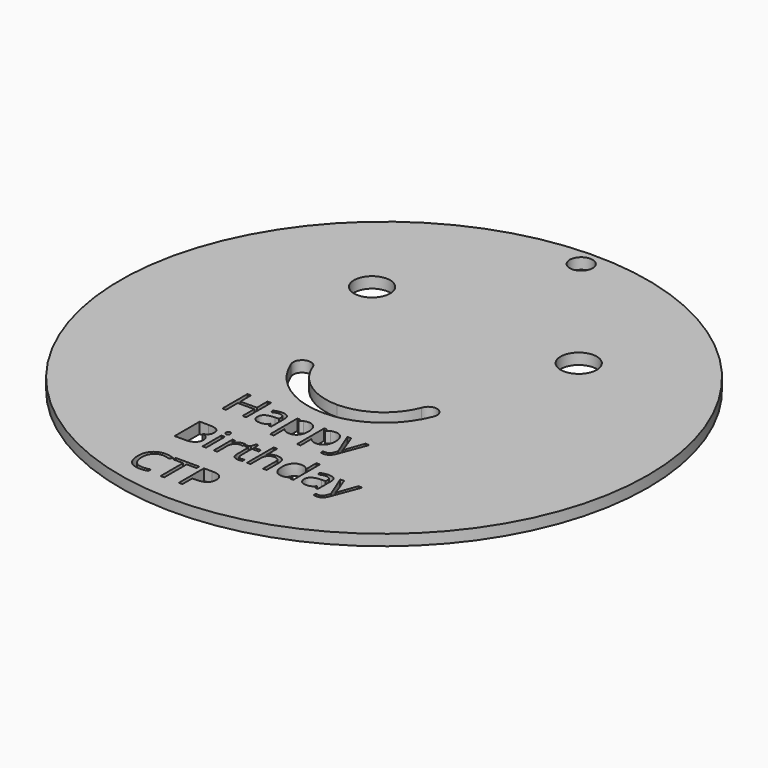
from build123d import *

# Parameters (mm, degrees)
F0_R     = 76.2
F0_W     = 1.0266422647
F0_H     = 6.7750477006
F0_R_2   = 5.2199295035
F0_R_3   = 3.304123166
F1_DEPTH = 3.175


with BuildPart() as f1:
    # F0 (on Top) → F1 (new body)
    with BuildSketch(Plane.XY):
        Circle(F0_R)
        with BuildLine():
            add(Edge.make_bspline(
                [(-13.1552634243, -61.2039017172), (-14.181905689, -60.7232195008), (-15.2085479537, -60.7232195008)],
                knots=[0, 0, 0, 1, 1, 1], degree=2))
            add(Edge.make_bspline(
                [(-15.2085479537, -60.7232195008), (-16.6980693898, -60.7232195008), (-17.5605280168, -61.7152447335)],
                knots=[0, 0, 0, 1, 1, 1], degree=2))
            add(Edge.make_bspline(
                [(-17.5605280168, -61.7152447335), (-18.4229866438, -62.7072699661), (-18.4229866438, -64.4321872201)],
                knots=[0, 0, 0, 1, 1, 1], degree=2))
            add(Edge.make_bspline(
                [(-18.4229866438, -64.4321872201), (-18.4229866438, -66.2045792609), (-17.5911888166, -67.1728671002)],
                knots=[0, 0, 0, 1, 1, 1], degree=2))
            add(Edge.make_bspline(
                [(-17.5911888166, -67.1728671002), (-16.7593909894, -68.1411549394), (-15.2204166504, -68.1411549394)],
                knots=[0, 0, 0, 1, 1, 1], degree=2))
            add(Edge.make_bspline(
                [(-15.2204166504, -68.1411549394), (-14.2748771465, -68.1411549394), (-13.0622919668, -67.8009189673)],
                knots=[0, 0, 0, 1, 1, 1], degree=2))
            Line((-13.0622919668, -67.8009189673), (-13.0622919668, -68.7207429617))
            add(Edge.make_bspline(
                [(-13.0622919668, -68.7207429617), (-14.0018971224, -69.0748257467), (-15.3806440559, -69.0748257467)],
                knots=[0, 0, 0, 1, 1, 1], degree=2))
            add(Edge.make_bspline(
                [(-15.3806440559, -69.0748257467), (-17.3765632179, -69.0748257467), (-18.4615599081, -67.862240567)],
                knots=[0, 0, 0, 1, 1, 1], degree=2))
            add(Edge.make_bspline(
                [(-18.4615599081, -67.862240567), (-19.5465565983, -66.6496553873), (-19.5465565983, -64.4183404073)],
                knots=[0, 0, 0, 1, 1, 1], degree=2))
            add(Edge.make_bspline(
                [(-19.5465565983, -64.4183404073), (-19.5465565983, -63.0217904287), (-19.0243339434, -61.9714107706)],
                knots=[0, 0, 0, 1, 1, 1], degree=2))
            add(Edge.make_bspline(
                [(-19.0243339434, -61.9714107706), (-18.5021112885, -60.9210311125), (-17.5160204042, -60.3523227289)],
                knots=[0, 0, 0, 1, 1, 1], degree=2))
            add(Edge.make_bspline(
                [(-17.5160204042, -60.3523227289), (-16.5299295199, -59.7836143452), (-15.1947011409, -59.7836143452)],
                knots=[0, 0, 0, 1, 1, 1], degree=2))
            add(Edge.make_bspline(
                [(-15.1947011409, -59.7836143452), (-13.7744137689, -59.7836143452), (-12.710187298, -60.3018807679)],
                knots=[0, 0, 0, 1, 1, 1], degree=2))
            Line((-12.710187298, -60.3018807679), (-13.1552634243, -61.2039017172))
        make_face(mode=Mode.SUBTRACT)
        Polygon((-8.3088789377, -60.8458627001), (-8.3088789377, -68.9502044313), (-9.3592585958, -68.9502044313), (-9.3592585958, -60.8458627001), (-12.2215926171, -60.8458627001), (-12.2215926171, -59.9121918928), (-5.4465449165, -59.9121918928), (-5.4465449165, -60.8458627001), align=None, mode=Mode.SUBTRACT)
        with BuildLine():
            add(Edge.make_bspline(
                [(-1.7415334294, -59.9121918928), (1.6450013629, -59.9121918928), (1.6450013629, -62.5450644445)],
                knots=[0, 0, 0, 1, 1, 1], degree=2))
            add(Edge.make_bspline(
                [(1.6450013629, -62.5450644445), (1.6450013629, -63.9178770297), (0.7083633815, -64.6567033994)],
                knots=[0, 0, 0, 1, 1, 1], degree=2))
            add(Edge.make_bspline(
                [(0.7083633815, -64.6567033994), (-0.2282745999, -65.3955297691), (-1.970994899, -65.3955297691)],
                knots=[0, 0, 0, 1, 1, 1], degree=2))
            Line((-1.970994899, -65.3955297691), (-3.0352213699, -65.3955297691))
            Line((-3.0352213699, -65.3955297691), (-3.0352213699, -68.9502044313))
            Line((-3.0352213699, -68.9502044313), (-4.085601028, -68.9502044313))
            Line((-4.085601028, -68.9502044313), (-4.085601028, -59.9121918928))
            Line((-4.085601028, -59.9121918928), (-1.7415334294, -59.9121918928))
        make_face(mode=Mode.SUBTRACT)
        with Locations((-10.5154674662, -48.3451578988)):
            Rectangle(F0_W, F0_H, mode=Mode.SUBTRACT)
        with BuildLine():
            add(Edge.make_bspline(
                [(-5.9034897395, -45.1920408084), (-5.371376504, -44.8330127331), (-4.7344231144, -44.8330127331)],
                knots=[0, 0, 0, 1, 1, 1], degree=2))
            add(Edge.make_bspline(
                [(-4.7344231144, -44.8330127331), (-4.2834126397, -44.8330127331), (-3.9253736225, -44.9081811456)],
                knots=[0, 0, 0, 1, 1, 1], degree=2))
            Line((-3.9253736225, -44.9081811456), (-4.0677979829, -45.8596549979))
            add(Edge.make_bspline(
                [(-4.0677979829, -45.8596549979), (-4.4871585997, -45.7666835404), (-4.8095915268, -45.7666835404)],
                knots=[0, 0, 0, 1, 1, 1], degree=2))
            add(Edge.make_bspline(
                [(-4.8095915268, -45.7666835404), (-5.6324878315, -45.7666835404), (-6.216032086, -46.4342977298)],
                knots=[0, 0, 0, 1, 1, 1], degree=2))
            add(Edge.make_bspline(
                [(-6.216032086, -46.4342977298), (-6.7995763405, -47.1019119193), (-6.7995763405, -48.0969043262)],
                knots=[0, 0, 0, 1, 1, 1], degree=2))
            Line((-6.7995763405, -48.0969043262), (-6.7995763405, -51.7326817492))
            Line((-6.7995763405, -51.7326817492), (-7.8262186052, -51.7326817492))
            Line((-7.8262186052, -51.7326817492), (-7.8262186052, -44.9576340485))
            Line((-7.8262186052, -44.9576340485), (-6.9795849071, -44.9576340485))
            Line((-6.9795849071, -44.9576340485), (-6.8608979401, -46.2117596667))
            Line((-6.8608979401, -46.2117596667), (-6.8114450372, -46.2117596667))
            add(Edge.make_bspline(
                [(-6.8114450372, -46.2117596667), (-6.435602975, -45.5510688836), (-5.9034897395, -45.1920408084)],
                knots=[0, 0, 0, 1, 1, 1], degree=2))
        make_face(mode=Mode.SUBTRACT)
        with BuildLine():
            Line((-19.0777430785, -51.7326817492), (-19.0777430785, -42.6946692107))
            Line((-19.0777430785, -42.6946692107), (-16.5239951715, -42.6946692107))
            add(Edge.make_bspline(
                [(-16.5239951715, -42.6946692107), (-14.7258876212, -42.6946692107), (-13.9217834196, -43.2327167945)],
                knots=[0, 0, 0, 1, 1, 1], degree=2))
            add(Edge.make_bspline(
                [(-13.9217834196, -43.2327167945), (-13.1176792181, -43.7707643783), (-13.1176792181, -44.931918539)],
                knots=[0, 0, 0, 1, 1, 1], degree=2))
            add(Edge.make_bspline(
                [(-13.1176792181, -44.931918539), (-13.1176792181, -45.7370117986), (-13.5657225186, -46.2592344535)],
                knots=[0, 0, 0, 1, 1, 1], degree=2))
            add(Edge.make_bspline(
                [(-13.5657225186, -46.2592344535), (-14.0137658191, -46.7814571084), (-14.87424633, -46.9357501655)],
                knots=[0, 0, 0, 1, 1, 1], degree=2))
            Line((-14.87424633, -46.9357501655), (-14.87424633, -46.9970717651))
            add(Edge.make_bspline(
                [(-14.87424633, -46.9970717651), (-12.8150274522, -47.3491764339), (-12.8150274522, -49.1611307971)],
                knots=[0, 0, 0, 1, 1, 1], degree=2))
            add(Edge.make_bspline(
                [(-12.8150274522, -49.1611307971), (-12.8150274522, -50.3717378607), (-13.6339675246, -51.0522098049)],
                knots=[0, 0, 0, 1, 1, 1], degree=2))
            add(Edge.make_bspline(
                [(-13.6339675246, -51.0522098049), (-14.4529075971, -51.7326817492), (-15.9246259881, -51.7326817492)],
                knots=[0, 0, 0, 1, 1, 1], degree=2))
            Line((-15.9246259881, -51.7326817492), (-19.0777430785, -51.7326817492))
        make_face(mode=Mode.SUBTRACT)
        with BuildLine():
            add(Edge.make_bspline(
                [(-10.9427405475, -43.6382305985), (-11.1158257077, -43.4681126124), (-11.1158257077, -43.121942292)],
                knots=[0, 0, 0, 1, 1, 1], degree=2))
            add(Edge.make_bspline(
                [(-11.1158257077, -43.121942292), (-11.1158257077, -42.7698376231), (-10.9427405475, -42.6056539854)],
                knots=[0, 0, 0, 1, 1, 1], degree=2))
            add(Edge.make_bspline(
                [(-10.9427405475, -42.6056539854), (-10.7696553873, -42.4414703477), (-10.5085440598, -42.4414703477)],
                knots=[0, 0, 0, 1, 1, 1], degree=2))
            add(Edge.make_bspline(
                [(-10.5085440598, -42.4414703477), (-10.2612795452, -42.4414703477), (-10.0822600366, -42.6086211596)],
                knots=[0, 0, 0, 1, 1, 1], degree=2))
            add(Edge.make_bspline(
                [(-10.0822600366, -42.6086211596), (-9.903240528, -42.7757719715), (-9.903240528, -43.121942292)],
                knots=[0, 0, 0, 1, 1, 1], degree=2))
            add(Edge.make_bspline(
                [(-9.903240528, -43.121942292), (-9.903240528, -43.4681126124), (-10.0822600366, -43.6382305985)],
                knots=[0, 0, 0, 1, 1, 1], degree=2))
            add(Edge.make_bspline(
                [(-10.0822600366, -43.6382305985), (-10.2612795452, -43.8083485846), (-10.5085440598, -43.8083485846)],
                knots=[0, 0, 0, 1, 1, 1], degree=2))
            add(Edge.make_bspline(
                [(-10.5085440598, -43.8083485846), (-10.7696553873, -43.8083485846), (-10.9427405475, -43.6382305985)],
                knots=[0, 0, 0, 1, 1, 1], degree=2))
        make_face(mode=Mode.SUBTRACT)
        with BuildLine():
            add(Edge.make_bspline(
                [(-1.2667855613, -50.681313033), (-0.9760024921, -51.0086912503), (-0.4696047662, -51.0086912503)],
                knots=[0, 0, 0, 1, 1, 1], degree=2))
            add(Edge.make_bspline(
                [(-0.4696047662, -51.0086912503), (-0.196624742, -51.0086912503), (0.0565741209, -50.969128928)],
                knots=[0, 0, 0, 1, 1, 1], degree=2))
            add(Edge.make_bspline(
                [(0.0565741209, -50.969128928), (0.3097729839, -50.9295666057), (0.4581316927, -50.8860480511)],
                knots=[0, 0, 0, 1, 1, 1], degree=2))
            Line((0.4581316927, -50.8860480511), (0.4581316927, -51.6713601495))
            add(Edge.make_bspline(
                [(0.4581316927, -51.6713601495), (0.2919699389, -51.7504847942), (-0.0324411043, -51.8038939294)],
                knots=[0, 0, 0, 1, 1, 1], degree=2))
            add(Edge.make_bspline(
                [(-0.0324411043, -51.8038939294), (-0.3568521475, -51.8573030645), (-0.6179634749, -51.8573030645)],
                knots=[0, 0, 0, 1, 1, 1], degree=2))
            add(Edge.make_bspline(
                [(-0.6179634749, -51.8573030645), (-2.5822327791, -51.8573030645), (-2.5822327791, -49.7862154901)],
                knots=[0, 0, 0, 1, 1, 1], degree=2))
            Line((-2.5822327791, -49.7862154901), (-2.5822327791, -45.7548148437))
            Line((-2.5822327791, -45.7548148437), (-3.5534877925, -45.7548148437))
            Line((-3.5534877925, -45.7548148437), (-3.5534877925, -45.2602858144))
            Line((-3.5534877925, -45.2602858144), (-2.5822327791, -44.8330127331))
            Line((-2.5822327791, -44.8330127331), (-2.1510034656, -43.3870098516))
            Line((-2.1510034656, -43.3870098516), (-1.5575686305, -43.3870098516))
            Line((-1.5575686305, -43.3870098516), (-1.5575686305, -44.9576340485))
            Line((-1.5575686305, -44.9576340485), (0.4086787898, -44.9576340485))
            Line((0.4086787898, -44.9576340485), (0.4086787898, -45.7548148437))
            Line((0.4086787898, -45.7548148437), (-1.5575686305, -45.7548148437))
            Line((-1.5575686305, -45.7548148437), (-1.5575686305, -49.7426969355))
            add(Edge.make_bspline(
                [(-1.5575686305, -49.7426969355), (-1.5575686305, -50.3539348156), (-1.2667855613, -50.681313033)],
                knots=[0, 0, 0, 1, 1, 1], degree=2))
        make_face(mode=Mode.SUBTRACT)
        Polygon((-12.2156582688, -25.4771465286), (-12.2156582688, -34.515159067), (-13.2660379269, -34.515159067), (-13.2660379269, -30.2622094155), (-18.0273634204, -30.2622094155), (-18.0273634204, -34.515159067), (-19.0777430785, -34.515159067), (-19.0777430785, -25.4771465286), (-18.0273634204, -25.4771465286), (-18.0273634204, -29.32260426), (-13.2660379269, -29.32260426), (-13.2660379269, -25.4771465286), align=None, mode=Mode.SUBTRACT)
        with BuildLine():
            Line((-4.9638845839, -34.515159067), (-5.725459289, -34.515159067))
            Line((-5.725459289, -34.515159067), (-5.929205249, -33.5498384019))
            Line((-5.929205249, -33.5498384019), (-5.9786581519, -33.5498384019))
            add(Edge.make_bspline(
                [(-5.9786581519, -33.5498384019), (-6.4850558779, -34.1867917916), (-6.9884864297, -34.413286087)],
                knots=[0, 0, 0, 1, 1, 1], degree=2))
            add(Edge.make_bspline(
                [(-6.9884864297, -34.413286087), (-7.4919169814, -34.6397803824), (-8.2475573381, -34.6397803824)],
                knots=[0, 0, 0, 1, 1, 1], degree=2))
            add(Edge.make_bspline(
                [(-8.2475573381, -34.6397803824), (-9.2544184416, -34.6397803824), (-9.8260939995, -34.1195358436)],
                knots=[0, 0, 0, 1, 1, 1], degree=2))
            add(Edge.make_bspline(
                [(-9.8260939995, -34.1195358436), (-10.3977695573, -33.5992913049), (-10.3977695573, -32.6418831042)],
                knots=[0, 0, 0, 1, 1, 1], degree=2))
            add(Edge.make_bspline(
                [(-10.3977695573, -32.6418831042), (-10.3977695573, -30.5905766909), (-7.1160749192, -30.4916708851)],
                knots=[0, 0, 0, 1, 1, 1], degree=2))
            Line((-7.1160749192, -30.4916708851), (-5.9667894552, -30.4540866789))
            Line((-5.9667894552, -30.4540866789), (-5.9667894552, -30.032747946))
            add(Edge.make_bspline(
                [(-5.9667894552, -30.032747946), (-5.9667894552, -29.2355671508), (-6.3090035435, -28.8557688564)],
                knots=[0, 0, 0, 1, 1, 1], degree=2))
            add(Edge.make_bspline(
                [(-6.3090035435, -28.8557688564), (-6.6512176317, -28.4759705619), (-7.4068579884, -28.4759705619)],
                knots=[0, 0, 0, 1, 1, 1], degree=2))
            add(Edge.make_bspline(
                [(-7.4068579884, -28.4759705619), (-8.2534916865, -28.4759705619), (-9.3216743896, -28.9942369845)],
                knots=[0, 0, 0, 1, 1, 1], degree=2))
            Line((-9.3216743896, -28.9942369845), (-9.6381729683, -28.2089248861))
            add(Edge.make_bspline(
                [(-9.6381729683, -28.2089248861), (-9.1377095907, -27.9379229781), (-8.5413075815, -27.783629921)],
                knots=[0, 0, 0, 1, 1, 1], degree=2))
            add(Edge.make_bspline(
                [(-8.5413075815, -27.783629921), (-7.9449055722, -27.6293368638), (-7.3435582727, -27.6293368638)],
                knots=[0, 0, 0, 1, 1, 1], degree=2))
            add(Edge.make_bspline(
                [(-7.3435582727, -27.6293368638), (-6.1329512091, -27.6293368638), (-5.5484178965, -28.1663953896)],
                knots=[0, 0, 0, 1, 1, 1], degree=2))
            add(Edge.make_bspline(
                [(-5.5484178965, -28.1663953896), (-4.9638845839, -28.7034539153), (-4.9638845839, -29.8903235855)],
                knots=[0, 0, 0, 1, 1, 1], degree=2))
            Line((-4.9638845839, -29.8903235855), (-4.9638845839, -34.515159067))
        make_face(mode=Mode.SUBTRACT)
        with BuildLine():
            Line((7.4745095596, -51.7326817492), (6.4478672949, -51.7326817492))
            Line((6.4478672949, -51.7326817492), (6.4478672949, -47.3491764339))
            add(Edge.make_bspline(
                [(6.4478672949, -47.3491764339), (6.4478672949, -46.522323897), (6.0710361746, -46.1138429189)],
                knots=[0, 0, 0, 1, 1, 1], degree=2))
            add(Edge.make_bspline(
                [(6.0710361746, -46.1138429189), (5.6942050543, -45.7053619407), (4.8891117947, -45.7053619407)],
                knots=[0, 0, 0, 1, 1, 1], degree=2))
            add(Edge.make_bspline(
                [(4.8891117947, -45.7053619407), (3.8209290915, -45.7053619407), (3.3293672365, -46.2869280791)],
                knots=[0, 0, 0, 1, 1, 1], degree=2))
            add(Edge.make_bspline(
                [(3.3293672365, -46.2869280791), (2.8378053814, -46.8684942175), (2.8378053814, -48.1898757837)],
                knots=[0, 0, 0, 1, 1, 1], degree=2))
            Line((2.8378053814, -48.1898757837), (2.8378053814, -51.7326817492))
            Line((2.8378053814, -51.7326817492), (1.8111631167, -51.7326817492))
            Line((1.8111631167, -51.7326817492), (1.8111631167, -42.1131030723))
            Line((1.8111631167, -42.1131030723), (2.8378053814, -42.1131030723))
            Line((2.8378053814, -42.1131030723), (2.8378053814, -45.0248899965))
            add(Edge.make_bspline(
                [(2.8378053814, -45.0248899965), (2.8378053814, -45.5510688836), (2.7883524785, -45.8972392041)],
                knots=[0, 0, 0, 1, 1, 1], degree=2))
            Line((2.7883524785, -45.8972392041), (2.8496740781, -45.8972392041))
            add(Edge.make_bspline(
                [(2.8496740781, -45.8972392041), (3.152325844, -45.4086445232), (3.7121327051, -45.1277520346)],
                knots=[0, 0, 0, 1, 1, 1], degree=2))
            add(Edge.make_bspline(
                [(3.7121327051, -45.1277520346), (4.2719395662, -44.846859546), (4.9880176006, -44.846859546)],
                knots=[0, 0, 0, 1, 1, 1], degree=2))
            add(Edge.make_bspline(
                [(4.9880176006, -44.846859546), (6.230274522, -44.846859546), (6.8523920408, -45.4373272069)],
                knots=[0, 0, 0, 1, 1, 1], degree=2))
            add(Edge.make_bspline(
                [(6.8523920408, -45.4373272069), (7.4745095596, -46.0277948678), (7.4745095596, -47.3135703438)],
                knots=[0, 0, 0, 1, 1, 1], degree=2))
            Line((7.4745095596, -47.3135703438), (7.4745095596, -51.7326817492))
        make_face(mode=Mode.SUBTRACT)
        with BuildLine():
            Line((14.3286819049, -51.7326817492), (14.1921918928, -50.8247264515))
            Line((14.1921918928, -50.8247264515), (14.1368046416, -50.8247264515))
            add(Edge.make_bspline(
                [(14.1368046416, -50.8247264515), (13.4266609556, -51.8573030645), (12.0103298158, -51.8573030645)],
                knots=[0, 0, 0, 1, 1, 1], degree=2))
            add(Edge.make_bspline(
                [(12.0103298158, -51.8573030645), (10.6810357852, -51.8573030645), (9.9422094155, -50.9483587088)],
                knots=[0, 0, 0, 1, 1, 1], degree=2))
            add(Edge.make_bspline(
                [(9.9422094155, -50.9483587088), (9.2033830458, -50.039414353), (9.2033830458, -48.3639500019)],
                knots=[0, 0, 0, 1, 1, 1], degree=2))
            add(Edge.make_bspline(
                [(9.2033830458, -48.3639500019), (9.2033830458, -46.6884856509), (9.9451765897, -45.760749192)],
                knots=[0, 0, 0, 1, 1, 1], degree=2))
            add(Edge.make_bspline(
                [(9.9451765897, -45.760749192), (10.6869701336, -44.8330127331), (12.0103298158, -44.8330127331)],
                knots=[0, 0, 0, 1, 1, 1], degree=2))
            add(Edge.make_bspline(
                [(12.0103298158, -44.8330127331), (13.3890767493, -44.8330127331), (14.1249359449, -45.8359176045)],
                knots=[0, 0, 0, 1, 1, 1], degree=2))
            Line((14.1249359449, -45.8359176045), (14.2060387057, -45.8359176045))
            Line((14.2060387057, -45.8359176045), (14.1625201511, -45.3473229236))
            Line((14.1625201511, -45.3473229236), (14.1368046416, -44.8705969394))
            Line((14.1368046416, -44.8705969394), (14.1368046416, -42.1131030723))
            Line((14.1368046416, -42.1131030723), (15.1634469063, -42.1131030723))
            Line((15.1634469063, -42.1131030723), (15.1634469063, -51.7326817492))
            Line((15.1634469063, -51.7326817492), (14.3286819049, -51.7326817492))
        make_face(mode=Mode.SUBTRACT)
        with BuildLine():
            Line((22.2668618823, -51.7326817492), (21.5052871773, -51.7326817492))
            Line((21.5052871773, -51.7326817492), (21.3015412172, -50.7673610841))
            Line((21.3015412172, -50.7673610841), (21.2520883143, -50.7673610841))
            add(Edge.make_bspline(
                [(21.2520883143, -50.7673610841), (20.7456905884, -51.4043144737), (20.2422600366, -51.6308087691)],
                knots=[0, 0, 0, 1, 1, 1], degree=2))
            add(Edge.make_bspline(
                [(20.2422600366, -51.6308087691), (19.7388294848, -51.8573030645), (18.9831891281, -51.8573030645)],
                knots=[0, 0, 0, 1, 1, 1], degree=2))
            add(Edge.make_bspline(
                [(18.9831891281, -51.8573030645), (17.9763280246, -51.8573030645), (17.4046524668, -51.3370585258)],
                knots=[0, 0, 0, 1, 1, 1], degree=2))
            add(Edge.make_bspline(
                [(17.4046524668, -51.3370585258), (16.832976909, -50.816813987), (16.832976909, -49.8594057864)],
                knots=[0, 0, 0, 1, 1, 1], degree=2))
            add(Edge.make_bspline(
                [(16.832976909, -49.8594057864), (16.832976909, -47.8080993731), (20.1146715471, -47.7091935672)],
                knots=[0, 0, 0, 1, 1, 1], degree=2))
            Line((20.1146715471, -47.7091935672), (21.263957011, -47.671609361))
            Line((21.263957011, -47.671609361), (21.263957011, -47.2502706281))
            add(Edge.make_bspline(
                [(21.263957011, -47.2502706281), (21.263957011, -46.453089833), (20.9217429228, -46.0732915385)],
                knots=[0, 0, 0, 1, 1, 1], degree=2))
            add(Edge.make_bspline(
                [(20.9217429228, -46.0732915385), (20.5795288345, -45.693493244), (19.8238884779, -45.693493244)],
                knots=[0, 0, 0, 1, 1, 1], degree=2))
            add(Edge.make_bspline(
                [(19.8238884779, -45.693493244), (18.9772547798, -45.693493244), (17.9090720766, -46.2117596667)],
                knots=[0, 0, 0, 1, 1, 1], degree=2))
            Line((17.9090720766, -46.2117596667), (17.5925734979, -45.4264475682))
            add(Edge.make_bspline(
                [(17.5925734979, -45.4264475682), (18.0930368755, -45.1554456602), (18.6894388848, -45.0011526031)],
                knots=[0, 0, 0, 1, 1, 1], degree=2))
            add(Edge.make_bspline(
                [(18.6894388848, -45.0011526031), (19.285840894, -44.846859546), (19.8871881936, -44.846859546)],
                knots=[0, 0, 0, 1, 1, 1], degree=2))
            add(Edge.make_bspline(
                [(19.8871881936, -44.846859546), (21.0977952572, -44.846859546), (21.6823285698, -45.3839180717)],
                knots=[0, 0, 0, 1, 1, 1], degree=2))
            add(Edge.make_bspline(
                [(21.6823285698, -45.3839180717), (22.2668618823, -45.9209765975), (22.2668618823, -47.1078462677)],
                knots=[0, 0, 0, 1, 1, 1], degree=2))
            Line((22.2668618823, -47.1078462677), (22.2668618823, -51.7326817492))
        make_face(mode=Mode.SUBTRACT)
        with BuildLine():
            Line((26.0371512013, -51.7702659554), (23.3033947276, -44.9576340485))
            Line((23.3033947276, -44.9576340485), (24.4052054048, -44.9576340485))
            Line((24.4052054048, -44.9576340485), (25.8887924925, -48.820894825))
            add(Edge.make_bspline(
                [(25.8887924925, -48.820894825), (26.3754090573, -50.1442545072), (26.4940960243, -50.731754994)],
                knots=[0, 0, 0, 1, 1, 1], degree=2))
            Line((26.4940960243, -50.731754994), (26.5435489272, -50.731754994))
            add(Edge.make_bspline(
                [(26.5435489272, -50.731754994), (26.6226735719, -50.4152564152), (26.8798286671, -49.6517035941)],
                knots=[0, 0, 0, 1, 1, 1], degree=2))
            add(Edge.make_bspline(
                [(26.8798286671, -49.6517035941), (27.1369837623, -48.8881507729), (28.5592492504, -44.9576340485)],
                knots=[0, 0, 0, 1, 1, 1], degree=2))
            Line((28.5592492504, -44.9576340485), (29.6590818115, -44.9576340485))
            Line((29.6590818115, -44.9576340485), (26.7472948873, -52.6722869047))
            add(Edge.make_bspline(
                [(26.7472948873, -52.6722869047), (26.3140874577, -53.8156380203), (25.7364775515, -54.2953311787)],
                knots=[0, 0, 0, 1, 1, 1], degree=2))
            add(Edge.make_bspline(
                [(25.7364775515, -54.2953311787), (25.1588676453, -54.7750243371), (24.3181682956, -54.7750243371)],
                knots=[0, 0, 0, 1, 1, 1], degree=2))
            add(Edge.make_bspline(
                [(24.3181682956, -54.7750243371), (23.8473766598, -54.7750243371), (23.3904318368, -54.6682060667)],
                knots=[0, 0, 0, 1, 1, 1], degree=2))
            Line((23.3904318368, -54.6682060667), (23.3904318368, -53.8472878782))
            add(Edge.make_bspline(
                [(23.3904318368, -53.8472878782), (23.7306678089, -53.9204781745), (24.1500284257, -53.9204781745)],
                knots=[0, 0, 0, 1, 1, 1], degree=2))
            add(Edge.make_bspline(
                [(24.1500284257, -53.9204781745), (25.2083205483, -53.9204781745), (25.6593310229, -52.7336085043)],
                knots=[0, 0, 0, 1, 1, 1], degree=2))
            Line((25.6593310229, -52.7336085043), (26.0371512013, -51.7702659554))
        make_face(mode=Mode.SUBTRACT)
        with BuildLine():
            add(Edge.make_bspline(
                [(2.3699809197, -33.7150110977), (1.6252202017, -34.6397803824), (0.3018605195, -34.6397803824)],
                knots=[0, 0, 0, 1, 1, 1], degree=2))
            add(Edge.make_bspline(
                [(0.3018605195, -34.6397803824), (-0.3608083797, -34.6397803824), (-0.9077574861, -34.3954830419)],
                knots=[0, 0, 0, 1, 1, 1], degree=2))
            add(Edge.make_bspline(
                [(-0.9077574861, -34.3954830419), (-1.4547065924, -34.1511857015), (-1.8246143063, -33.6428098594)],
                knots=[0, 0, 0, 1, 1, 1], degree=2))
            Line((-1.8246143063, -33.6428098594), (-1.8997827187, -33.6428098594))
            add(Edge.make_bspline(
                [(-1.8997827187, -33.6428098594), (-1.8246143063, -34.2362446945), (-1.8246143063, -34.76835793)],
                knots=[0, 0, 0, 1, 1, 1], degree=2))
            Line((-1.8246143063, -34.76835793), (-1.8246143063, -37.5575016549))
            Line((-1.8246143063, -37.5575016549), (-2.851256571, -37.5575016549))
            Line((-2.851256571, -37.5575016549), (-2.851256571, -27.7401113664))
            Line((-2.851256571, -27.7401113664), (-2.0164915696, -27.7401113664))
            Line((-2.0164915696, -27.7401113664), (-1.8740672092, -28.6678478252))
            Line((-1.8740672092, -28.6678478252), (-1.8246143063, -28.6678478252))
            add(Edge.make_bspline(
                [(-1.8246143063, -28.6678478252), (-1.4289910829, -28.1100190803), (-0.9038012538, -27.8627545656)],
                knots=[0, 0, 0, 1, 1, 1], degree=2))
            add(Edge.make_bspline(
                [(-0.9038012538, -27.8627545656), (-0.3786114248, -27.615490051), (0.3018605195, -27.615490051)],
                knots=[0, 0, 0, 1, 1, 1], degree=2))
            add(Edge.make_bspline(
                [(0.3018605195, -27.615490051), (1.6489575951, -27.615490051), (2.3818496164, -28.5372921615)],
                knots=[0, 0, 0, 1, 1, 1], degree=2))
            add(Edge.make_bspline(
                [(2.3818496164, -28.5372921615), (3.1147416378, -29.459094272), (3.1147416378, -31.1207118103)],
                knots=[0, 0, 0, 1, 1, 1], degree=2))
            add(Edge.make_bspline(
                [(3.1147416378, -31.1207118103), (3.1147416378, -32.790241813), (2.3699809197, -33.7150110977)],
                knots=[0, 0, 0, 1, 1, 1], degree=2))
        make_face(mode=Mode.SUBTRACT)
        with BuildLine():
            add(Edge.make_bspline(
                [(10.1281523305, -33.7150110977), (9.3833916125, -34.6397803824), (8.0600319302, -34.6397803824)],
                knots=[0, 0, 0, 1, 1, 1], degree=2))
            add(Edge.make_bspline(
                [(8.0600319302, -34.6397803824), (7.397363031, -34.6397803824), (6.8504139247, -34.3954830419)],
                knots=[0, 0, 0, 1, 1, 1], degree=2))
            add(Edge.make_bspline(
                [(6.8504139247, -34.3954830419), (6.3034648183, -34.1511857015), (5.9335571045, -33.6428098594)],
                knots=[0, 0, 0, 1, 1, 1], degree=2))
            Line((5.9335571045, -33.6428098594), (5.858388692, -33.6428098594))
            add(Edge.make_bspline(
                [(5.858388692, -33.6428098594), (5.9335571045, -34.2362446945), (5.9335571045, -34.76835793)],
                knots=[0, 0, 0, 1, 1, 1], degree=2))
            Line((5.9335571045, -34.76835793), (5.9335571045, -37.5575016549))
            Line((5.9335571045, -37.5575016549), (4.9069148398, -37.5575016549))
            Line((4.9069148398, -37.5575016549), (4.9069148398, -27.7401113664))
            Line((4.9069148398, -27.7401113664), (5.7416798411, -27.7401113664))
            Line((5.7416798411, -27.7401113664), (5.8841042015, -28.6678478252))
            Line((5.8841042015, -28.6678478252), (5.9335571045, -28.6678478252))
            add(Edge.make_bspline(
                [(5.9335571045, -28.6678478252), (6.3291803279, -28.1100190803), (6.8543701569, -27.8627545656)],
                knots=[0, 0, 0, 1, 1, 1], degree=2))
            add(Edge.make_bspline(
                [(6.8543701569, -27.8627545656), (7.379559986, -27.615490051), (8.0600319302, -27.615490051)],
                knots=[0, 0, 0, 1, 1, 1], degree=2))
            add(Edge.make_bspline(
                [(8.0600319302, -27.615490051), (9.4071290059, -27.615490051), (10.1400210272, -28.5372921615)],
                knots=[0, 0, 0, 1, 1, 1], degree=2))
            add(Edge.make_bspline(
                [(10.1400210272, -28.5372921615), (10.8729130486, -29.459094272), (10.8729130486, -31.1207118103)],
                knots=[0, 0, 0, 1, 1, 1], degree=2))
            add(Edge.make_bspline(
                [(10.8729130486, -31.1207118103), (10.8729130486, -32.790241813), (10.1281523305, -33.7150110977)],
                knots=[0, 0, 0, 1, 1, 1], degree=2))
        make_face(mode=Mode.SUBTRACT)
        with BuildLine():
            Line((14.3227475566, -34.5527432732), (11.5889910829, -27.7401113664))
            Line((11.5889910829, -27.7401113664), (12.6908017601, -27.7401113664))
            Line((12.6908017601, -27.7401113664), (14.1743888478, -31.6033721428))
            add(Edge.make_bspline(
                [(14.1743888478, -31.6033721428), (14.6610054126, -32.9267318251), (14.7796923796, -33.5142323118)],
                knots=[0, 0, 0, 1, 1, 1], degree=2))
            Line((14.7796923796, -33.5142323118), (14.8291452825, -33.5142323118))
            add(Edge.make_bspline(
                [(14.8291452825, -33.5142323118), (14.9082699272, -33.1977337331), (15.1654250224, -32.434180912)],
                knots=[0, 0, 0, 1, 1, 1], degree=2))
            add(Edge.make_bspline(
                [(15.1654250224, -32.434180912), (15.4225801176, -31.6706280908), (16.8448456057, -27.7401113664)],
                knots=[0, 0, 0, 1, 1, 1], degree=2))
            Line((16.8448456057, -27.7401113664), (17.9446781667, -27.7401113664))
            Line((17.9446781667, -27.7401113664), (15.0328912426, -35.4547642226))
            add(Edge.make_bspline(
                [(15.0328912426, -35.4547642226), (14.5996838129, -36.5981153382), (14.0220739068, -37.0778084966)],
                knots=[0, 0, 0, 1, 1, 1], degree=2))
            add(Edge.make_bspline(
                [(14.0220739068, -37.0778084966), (13.4444640006, -37.5575016549), (12.6037646509, -37.5575016549)],
                knots=[0, 0, 0, 1, 1, 1], degree=2))
            add(Edge.make_bspline(
                [(12.6037646509, -37.5575016549), (12.1329730151, -37.5575016549), (11.676028192, -37.4506833846)],
                knots=[0, 0, 0, 1, 1, 1], degree=2))
            Line((11.676028192, -37.4506833846), (11.676028192, -36.6297651961))
            add(Edge.make_bspline(
                [(11.676028192, -36.6297651961), (12.0162641642, -36.7029554924), (12.435624781, -36.7029554924)],
                knots=[0, 0, 0, 1, 1, 1], degree=2))
            add(Edge.make_bspline(
                [(12.435624781, -36.7029554924), (13.4939169035, -36.7029554924), (13.9449273782, -35.5160858222)],
                knots=[0, 0, 0, 1, 1, 1], degree=2))
            Line((13.9449273782, -35.5160858222), (14.3227475566, -34.5527432732))
        make_face(mode=Mode.SUBTRACT)
        with BuildLine():
            ThreePointArc((0, -21.991588294), (-12.3974898875, -18.1640359001), (-20.4795077443, -8.0137206241))
            ThreePointArc((-20.4795077443, -8.0137206241), (-19.1391930287, -4.4685947082), (-15.7487944393, -6.1625718928))
            ThreePointArc((-15.7487944393, -6.1625718928), (-9.5337017979, -13.9681906006), (0, -16.911588294))
            ThreePointArc((0, -16.911588294), (9.5337017979, -13.9681906006), (15.7487944393, -6.1625718928))
            ThreePointArc((15.7487944393, -6.1625718928), (19.1391930287, -4.4685947082), (20.4795077443, -8.0137206241))
            ThreePointArc((20.4795077443, -8.0137206241), (12.3974898875, -18.1640359001), (0, -21.991588294))
        make_face(mode=Mode.SUBTRACT)
        with Locations((-29.8356824311, 32.9489689349)):
            Circle(F0_R_2, mode=Mode.SUBTRACT)
        with Locations((29.8356824311, 32.9489689349)):
            Circle(F0_R_2, mode=Mode.SUBTRACT)
        with Locations((0, 71.12)):
            Circle(F0_R_3, mode=Mode.SUBTRACT)
    extrude(amount=F1_DEPTH)


solid = f1.part
